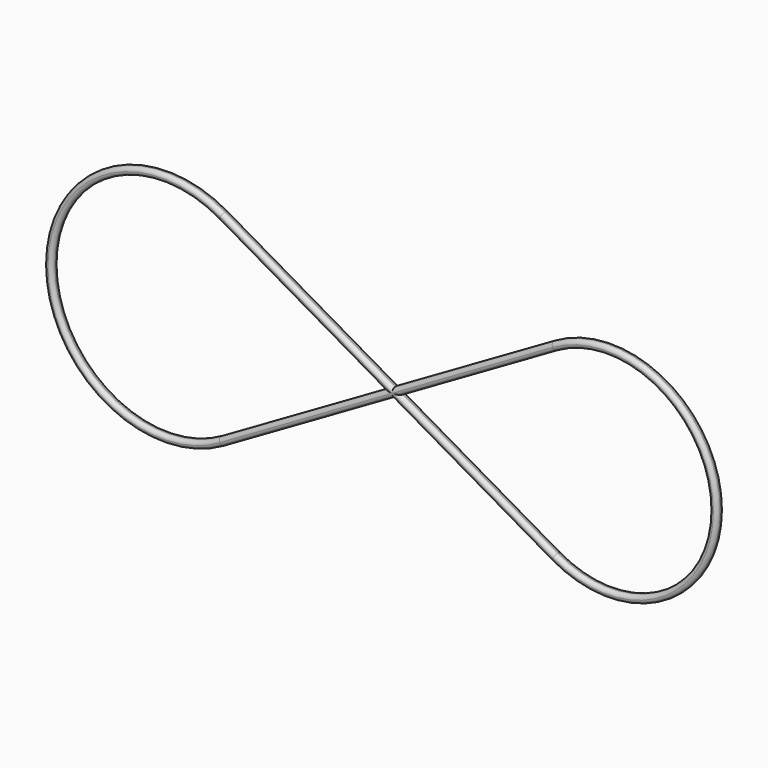
from build123d import *

# Parameters (mm, degrees)
F1_DEPTH = 0.55
F2_R     = 0.49999


# Not quite as in the source:
# - a fillet or chamfer is up to 0.001 mm smaller than in the source, because OpenCascade refuses the exact size


with BuildPart() as f1:
    # F0 (on Front) → F1 (new body, symmetric)
    with BuildSketch(Plane.XZ):
        with BuildLine():
            Line((1, -0.5773502692), (0, 0))
            Line((0, 0), (1, 0.5773502692))
            Line((1, 0.5773502692), (-21.1506350946, 13.3660254038))
            ThreePointArc((-21.1506350946, 13.3660254038), (-44.3012701892, 0), (-21.1506350946, -13.3660254038))
            Line((-21.1506350946, -13.3660254038), (1, -0.5773502692))
        make_face()
        with BuildLine():
            Line((0, 0), (-21.6506350946, -12.5))
            ThreePointArc((-21.6506350946, -12.5), (-43.3012701892, 0), (-21.6506350946, 12.5))
            Line((-21.6506350946, 12.5), (0, 0))
        make_face(mode=Mode.SUBTRACT)
        Polygon((1, 0.5773502692), (0, 0), (1, -0.5773502692), (2, 0), align=None)
        with BuildLine():
            Line((21.6506350946, 12.5), (1, 0.5773502692))
            Line((1, 0.5773502692), (2, 0))
            Line((2, 0), (1, -0.5773502692))
            Line((1, -0.5773502692), (21.6506350946, -12.5))
            ThreePointArc((21.6506350946, -12.5), (43.3012701892, 0), (21.6506350946, 12.5))
        make_face()
        with BuildLine():
            Line((22.1506350946, -11.6339745962), (2, 0))
            Line((2, 0), (22.1506350946, 11.6339745962))
            ThreePointArc((22.1506350946, 11.6339745962), (42.3012701892, 0), (22.1506350946, -11.6339745962))
        make_face(mode=Mode.SUBTRACT)
    extrude(amount=F1_DEPTH, both=True)

    # F2 (radius 0.5 in the source; OpenCascade refuses exactly that, so slightly less here)
    f2_edges = [f1.edges().sort_by_distance(p)[0] for p in [
        (-44.30127, -0.55, 0),
        (-10.075318, -0.55, -6.971688),
        (11.325318, -0.55, -6.538675),
        (43.30127, -0.55, 0),
        (11.325318, -0.55, 6.538675),
        (-10.075318, -0.55, 6.971688),
        (-10.825318, -0.55, 6.25),
        (-10.825318, -0.55, -6.25),
        (-43.30127, -0.55, 0),
        (12.075318, -0.55, 5.816987),
        (42.30127, -0.55, 0),
        (12.075318, -0.55, -5.816987),
        (-44.30127, 0.55, 0),
        (-10.075318, 0.55, -6.971688),
        (11.325318, 0.55, -6.538675),
        (43.30127, 0.55, 0),
        (11.325318, 0.55, 6.538675),
        (-10.075318, 0.55, 6.971688),
        (-10.825318, 0.55, 6.25),
        (-10.825318, 0.55, -6.25),
        (-43.30127, 0.55, 0),
        (12.075318, 0.55, 5.816987),
        (42.30127, 0.55, 0),
        (12.075318, 0.55, -5.816987),
    ]]
    fillet(f2_edges, radius=F2_R)


solid = f1.part
